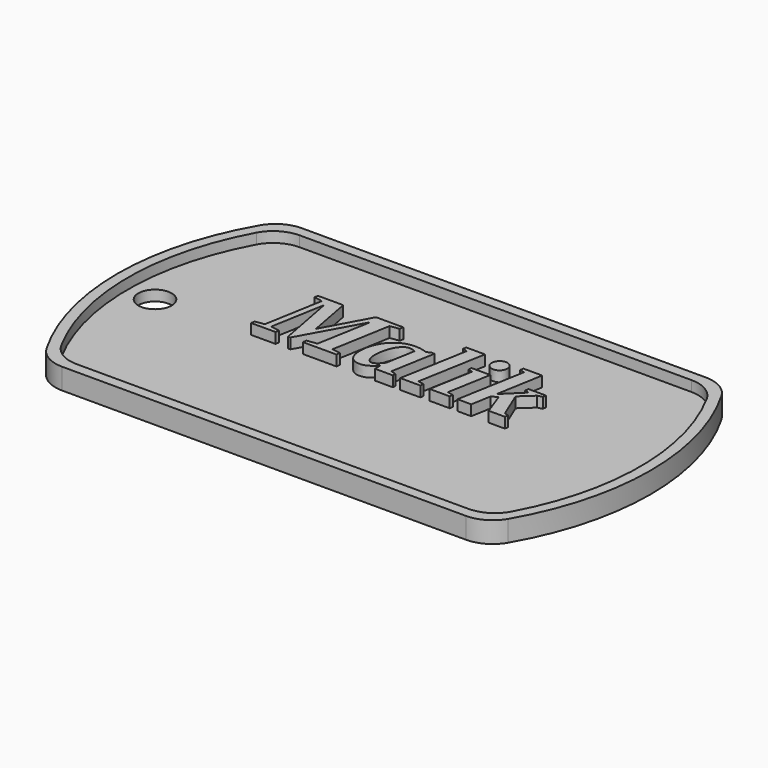
from build123d import *

# Parameters (mm, degrees)
F1_DEPTH     = 1
F3_DEPTH     = 1
F4_R         = 1.5875
F5_DEPTH     = 1
F6_TEXT_SIZE = 9.9742099539
F7_DEPTH     = 1


# Not quite as in the source:
# - Text() gives the source's letters only with a copy of the font that has no kerning and outlines rounded to 1/6400 em; it was checked with that copy


with BuildPart() as f1:
    # F0 (on Top) → F1 (new body)
    with BuildSketch(Plane.XY):
        with BuildLine():
            ThreePointArc((-19.2474145991, 14.2875), (-20.8349145991, 13.862130657), (-21.9970452561, 12.7))
            ThreePointArc((-21.9970452561, 12.7), (-25.4, 0), (-21.9970452561, -12.7))
            ThreePointArc((-21.9970452561, -12.7), (-20.8349145991, -13.862130657), (-19.2474145991, -14.2875))
            Line((-19.2474145991, -14.2875), (19.2474145991, -14.2875))
            ThreePointArc((19.2474145991, -14.2875), (20.8349145991, -13.862130657), (21.9970452561, -12.7))
            ThreePointArc((21.9970452561, -12.7), (25.4, 0), (21.9970452561, 12.7))
            ThreePointArc((21.9970452561, 12.7), (20.8349145991, 13.862130657), (19.2474145991, 14.2875))
            Line((19.2474145991, 14.2875), (-19.2474145991, 14.2875))
        make_face()
    extrude(amount=F1_DEPTH)

    # F2 (on face) → F3 (join)
    with BuildSketch(Plane.XY.offset(1)):
        with BuildLine():
            Line((19.2474145991, 14.2875), (-19.2474145991, 14.2875))
            ThreePointArc((-19.2474145991, 14.2875), (-20.8349145991, 13.862130657), (-21.9970452561, 12.7))
            ThreePointArc((-21.9970452561, 12.7), (-25.4, 0), (-21.9970452561, -12.7))
            ThreePointArc((-21.9970452561, -12.7), (-20.8349145991, -13.862130657), (-19.2474145991, -14.2875))
            Line((-19.2474145991, -14.2875), (19.2474145991, -14.2875))
            ThreePointArc((19.2474145991, -14.2875), (20.8349145991, -13.862130657), (21.9970452561, -12.7))
            ThreePointArc((21.9970452561, -12.7), (25.4, 0), (21.9970452561, 12.7))
            ThreePointArc((21.9970452561, 12.7), (20.8349145991, 13.862130657), (19.2474145991, 14.2875))
        make_face()
        with BuildLine():
            ThreePointArc((-21.4526124879, 11.6252061249), (-20.2856017842, 12.8404540819), (-18.6611352482, 13.2875))
            Line((-18.6611352482, 13.2875), (18.6611352482, 13.2875))
            ThreePointArc((18.6611352482, 13.2875), (20.2856017842, 12.8404540819), (21.4526124879, 11.6252061249))
            ThreePointArc((21.4526124879, 11.6252061249), (24.4, 0), (21.4526124879, -11.6252061249))
            ThreePointArc((21.4526124879, -11.6252061249), (20.2856017842, -12.8404540819), (18.6611352482, -13.2875))
            Line((18.6611352482, -13.2875), (-18.6611352482, -13.2875))
            ThreePointArc((-18.6611352482, -13.2875), (-20.2856017842, -12.8404540819), (-21.4526124879, -11.6252061249))
            ThreePointArc((-21.4526124879, -11.6252061249), (-24.4, 0), (-21.4526124879, 11.6252061249))
        make_face(mode=Mode.SUBTRACT)
    extrude(amount=F3_DEPTH)

    # F4 (on face) → F5 (cut)
    with BuildSketch(Plane.XY.offset(1)):
        with Locations((-21.821282804, 0)):
            Circle(F4_R)
    extrude(amount=-F5_DEPTH, mode=Mode.SUBTRACT)

    # F6 (on face) → F7 (join)
    with BuildSketch(Plane.XY.offset(1)):
        with Locations((-12.5308804898, 0)):
            Text('Malik', F6_TEXT_SIZE, font='Tinos', font_style=FontStyle.BOLDITALIC, text_align=(TextAlign.LEFT, TextAlign.BOTTOM))
    extrude(amount=F7_DEPTH)


solid = f1.part
